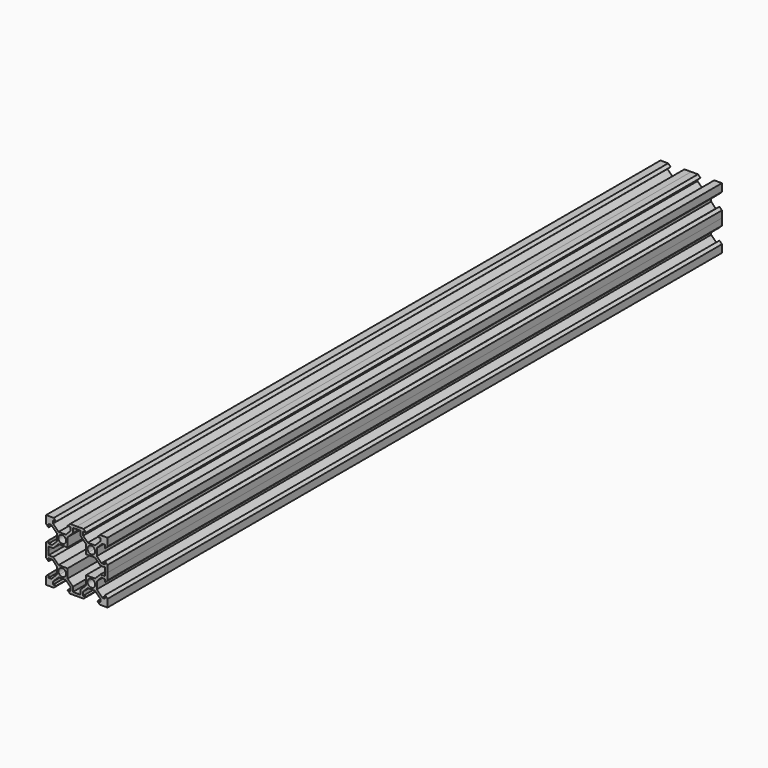
from build123d import *

# Parameters (mm, degrees)
F1_DEPTH        = 500
F1_COPIES_COUNT = 4


# Not quite as in the source:
# - a pattern or mirror of a feature is missing from the dataset's text; its kind, count and spacing are read off the source's solid


with BuildPart() as f1:
    # F0 (on Front) → F1 (new body)
    with BuildSketch(Plane.XZ):
        Polygon((-13, 11.8686291501), (-13, 13), (-20, 20), (-20, 15), (-18.4, 13.4), (-18.4, 15.4686291501), (-16.6, 15.4686291501), align=None)
        Polygon((-20, 20), (-13, 13), (-11.8686291501, 13), (-15.4686291501, 16.6), (-15.4686291501, 18.4), (-13.4, 18.4), (-15, 20), align=None)
        Polygon((-15.3372583002, 2.5313708499), (-11.8686291501, 6), (-13, 6), (-13, 7.1313708499), (-16, 4.1313708499), (-18.4, 4.1313708499), (-18.4, 6), (-20, 4.4), (-20, 0), (-18.4, 0), (-18.4, 2.5313708499), align=None)
        with BuildLine():
            Line((-11.8686291501, 6), (-6, 6))
            Line((-6, 6), (-7.732233047, 7.732233047))
            ThreePointArc((-7.732233047, 7.732233047), (-11.267766953, 7.732233047), (-11.267766953, 11.267766953))
            Line((-11.267766953, 11.267766953), (-13, 13))
            Line((-13, 13), (-13, 11.8686291501))
            Line((-13, 11.8686291501), (-13, 7.1313708499))
            Line((-13, 7.1313708499), (-13, 6))
            Line((-13, 6), (-11.8686291501, 6))
        make_face()
        with BuildLine():
            Line((-7.732233047, 7.732233047), (-6, 6))
            Line((-6, 6), (-6, 11.8686291501))
            Line((-6, 11.8686291501), (-6, 13))
            Line((-6, 13), (-7.1313708499, 13))
            Line((-7.1313708499, 13), (-11.8686291501, 13))
            Line((-11.8686291501, 13), (-13, 13))
            Line((-13, 13), (-11.267766953, 11.267766953))
            ThreePointArc((-11.267766953, 11.267766953), (-8.5432914191, 11.8096988313), (-7, 9.5))
            ThreePointArc((-7, 9.5), (-7.1903011687, 8.5432914191), (-7.732233047, 7.732233047))
        make_face()
        Polygon((-6, 13), (-6, 11.8686291501), (-2.5313708499, 15.3372583002), (-2.5313708499, 18.4), (0, 18.4), (0, 20), (-4.4, 20), (-6, 18.4), (-4.1313708499, 18.4), (-4.1313708499, 16), (-7.1313708499, 13), align=None)
    extrude(amount=F1_DEPTH)


with BuildPart() as f1_copies_1:
    # F1_copies: instance of F1
    add(f1.part.rotate(Axis((0, 0, 0), (0, 1, 0)), 1 * 360 / F1_COPIES_COUNT))


with BuildPart() as f1_copies_2:
    # F1_copies: instance of F1
    add(f1.part.rotate(Axis((0, 0, 0), (0, 1, 0)), 2 * 360 / F1_COPIES_COUNT))


with BuildPart() as f1_copies_3:
    # F1_copies: instance of F1
    add(f1.part.rotate(Axis((0, 0, 0), (0, 1, 0)), 3 * 360 / F1_COPIES_COUNT))


solid = Compound([f1.part, f1_copies_1.part, f1_copies_2.part, f1_copies_3.part])
